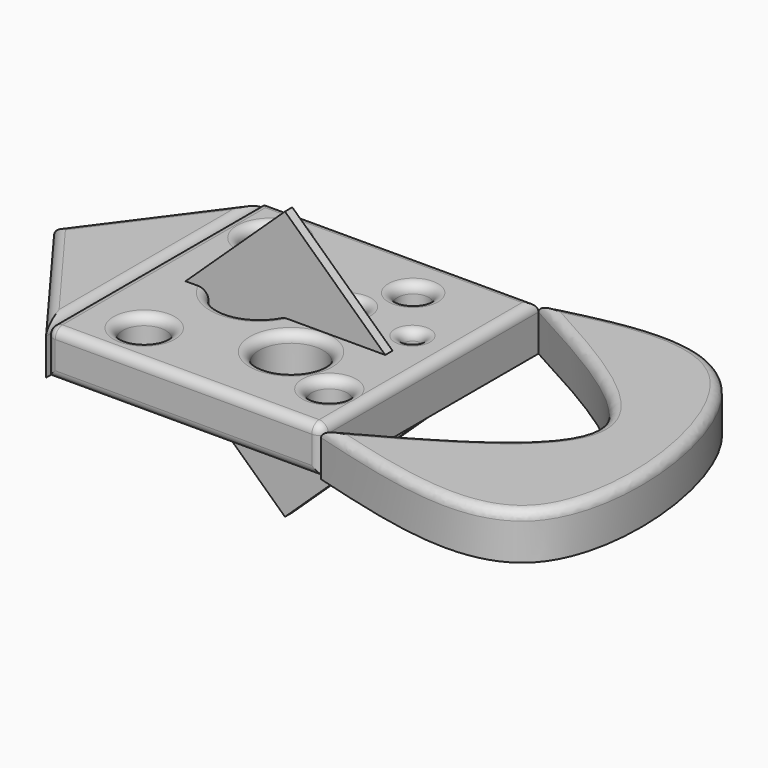
from build123d import *

# Parameters (mm, degrees)
F0_W         = 152.6045948267
F0_H         = 150.9183645248
F0_R         = 11.9309586608
F0_R_2       = 9.9286899081
F0_R_3       = 17.7906163948
F0_R_4       = 22.2629786526
F0_R_5       = 13.4964962962
F0_R_6       = 8.1874520601
F0_R_7       = 4.7131794668
F0_R_8       = 8.6804433709
F1_DEPTH     = 25.4
F3_DEPTH     = 25.4
F5_DEPTH     = 5.08
F6_T1_DEPTH  = 33.02
F6_T3_DEPTH  = 178.0045948267
F6_T5_DEPTH  = 142.4445948267
F6_T7_DEPTH  = 158.5383645248
F6_S11_W     = 5.08
F6_S11_H     = 5.08
F6_T12_DEPTH = 5.08
F6_S17_W     = 5.08
F6_S17_H     = 5.08
F6_T18_DEPTH = 5.08
F7_R         = 5.08
F8_R         = 5.08


# Not quite as in the source:
# - a fillet or chamfer that OpenCascade refuses, or shapes differently, is made with other operations: its cross-section is extruded or revolved along the edge and cut away or added


with BuildPart() as f1:
    # F0 (on Top) → F1 (new body)
    with BuildSketch(Plane.XY):
        Rectangle(F0_W, F0_H)
        with Locations((-41.7344048619, -50.5871586502)):
            Circle(F0_R, mode=Mode.SUBTRACT)
        with Locations((56.7151419818, -45.2293604612)):
            Circle(F0_R_2, mode=Mode.SUBTRACT)
        with Locations((21.9211075455, -28.2444972545)):
            Circle(F0_R_3, mode=Mode.SUBTRACT)
        with Locations((-23.6073378474, 6.744956132)):
            Circle(F0_R_4, mode=Mode.SUBTRACT)
        with Locations((-51.8518351018, 49.7440397739)):
            Circle(F0_R_5, mode=Mode.SUBTRACT)
        with Locations((14.5029760897, 19.8888368905)):
            Circle(F0_R_6, mode=Mode.SUBTRACT)
        with Locations((53.5380840302, 16.4408273995)):
            Circle(F0_R_7, mode=Mode.SUBTRACT)
        with Locations((28.6660604179, 48.0578020215)):
            Circle(F0_R_8, mode=Mode.SUBTRACT)
    extrude(amount=F1_DEPTH)

    # F6: fillet of radius 5.08 on 15 edges, made by hand

    # F6_s2 → F6_t1 (cut)
    with BuildSketch(Plane.XY.offset(-12.7)):
        with BuildLine():
            ThreePointArc((-76.3022974133, -70.3791822624), (-74.8143998618, -73.9712847108), (-71.2222974133, -75.4591822624))
            Line((-71.2222974133, -75.4591822624), (-76.3022974133, -75.4591822624))
            Line((-76.3022974133, -75.4591822624), (-76.3022974133, -70.3791822624))
        make_face()
        with BuildLine():
            ThreePointArc((71.2222974133, -75.4591822624), (74.8143998618, -73.9712847108), (76.3022974133, -70.3791822624))
            Line((76.3022974133, -70.3791822624), (76.3022974133, -75.4591822624))
            Line((76.3022974133, -75.4591822624), (71.2222974133, -75.4591822624))
        make_face()
    extrude(amount=F6_T1_DEPTH, mode=Mode.SUBTRACT)

    # F6_s4 → F6_t3 (cut)
    with BuildSketch(Plane.YZ.offset(-89.0022974133)):
        with BuildLine():
            ThreePointArc((-75.4591822624, 5.08), (-73.9712847108, 1.4878975516), (-70.3791822624, 0))
            Line((-70.3791822624, 0), (-75.4591822624, 0))
            Line((-75.4591822624, 0), (-75.4591822624, 5.08))
        make_face()
        with BuildLine():
            ThreePointArc((75.4591822624, 20.32), (73.9712847108, 23.9121024484), (70.3791822624, 25.4))
            Line((70.3791822624, 25.4), (75.4591822624, 25.4))
            Line((75.4591822624, 25.4), (75.4591822624, 20.32))
        make_face()
    extrude(amount=F6_T3_DEPTH, mode=Mode.SUBTRACT)

    # F6_s6 → F6_t5 (cut)
    with BuildSketch(Plane.YZ.offset(-71.2222974133)):
        with BuildLine():
            ThreePointArc((-75.4591822624, 20.32), (-73.9712847108, 23.9121024484), (-70.3791822624, 25.4))
            Line((-70.3791822624, 25.4), (-75.4591822624, 25.4))
            Line((-75.4591822624, 25.4), (-75.4591822624, 20.32))
        make_face()
    extrude(amount=F6_T5_DEPTH, mode=Mode.SUBTRACT)

    # F6_s8 → F6_t7 (cut)
    with BuildSketch(Plane.XZ.offset(-88.1591822624)):
        with BuildLine():
            ThreePointArc((-76.3022974133, 20.32), (-74.8143998618, 23.9121024484), (-71.2222974133, 25.4))
            Line((-71.2222974133, 25.4), (-76.3022974133, 25.4))
            Line((-76.3022974133, 25.4), (-76.3022974133, 20.32))
        make_face()
        with BuildLine():
            ThreePointArc((76.3022974133, 20.32), (74.8143998618, 23.9121024484), (71.2222974133, 25.4))
            Line((71.2222974133, 25.4), (76.3022974133, 25.4))
            Line((76.3022974133, 25.4), (76.3022974133, 20.32))
        make_face()
    extrude(amount=F6_T7_DEPTH, mode=Mode.SUBTRACT)


with BuildPart() as f3:
    # F2 (on face) → F3 (new body)
    with BuildSketch(Plane.XY.offset(25.4)):
        Polygon((-76.3022974133, -75.4591822624), (-76.3022974133, 75.4591822624), (-132.2656422853, 0), align=None)
    extrude(amount=-F3_DEPTH)

    # F8
    f8_edges = [f3.edges().sort_by_distance(p)[0] for p in [
        (-76.302297, 0, 25.4),
        (-104.28397, 37.729591, 25.4),
        (-104.28397, -37.729591, 25.4),
    ]]
    fillet(f8_edges, radius=F8_R)


with BuildPart() as f3b:
    # F2 (on face) → F3, piece 2 (new body)
    with BuildSketch(Plane.XY.offset(25.4)):
        with BuildLine():
            add(Edge.make_bspline(
                [(76.3022974133, 75.4591822624), (116.4970383218, 85.8497470481), (203.7587624378, 108.4073895966), (233.5011205607, -119.9087985164), (127.2335971306, -89.8605415247), (76.3022974133, -75.4591822624)],
                knots=[0, 0, 0, 0, 0.3078121712, 0.6682521185, 1, 1, 1, 1], degree=3))
            add(Edge.make_bspline(
                [(76.3022974133, 75.4591822624), (122.6474307477, 50.3061215083), (215.3376974165, 0), (122.6474307477, -50.3061215083), (76.3022974133, -75.4591822624)],
                knots=[0, 0, 0, 0, 0.5, 1, 1, 1, 1], degree=3))
        make_face()
    extrude(amount=-F3_DEPTH)

    # F7
    f7_edges = [f3b.edges().sort_by_distance(p)[0] for p in [
        (212.260303, -10.111069, 25.4),
        (168.992564, 0, 25.4),
    ]]
    fillet(f7_edges, radius=F7_R)


with BuildPart() as f5:
    # F4 (on Front) → F5 (new body)
    with BuildSketch(Plane.XZ):
        Polygon((0, 77.4029865861), (-76.8501013517, 4.9759130925), (75.7443532348, 6.6345483065), align=None)
    extrude(amount=F5_DEPTH)


with BuildPart() as f5b:
    # F4 (on Front) → F5, piece 2 (new body)
    with BuildSketch(Plane.XZ):
        Polygon((76.1863735795, 0), (-76.8501013517, 0), (0, -71.8015458847), align=None)
    extrude(amount=F5_DEPTH)


with BuildPart() as f6_tool10:
    # F6_s11 → F6_t12 (new body)
    with BuildSketch(Plane.YZ.offset(-71.2222974133)):
        with Locations((-72.9191822624, 22.86)):
            Rectangle(F6_S11_W, F6_S11_H)
    extrude(amount=-F6_T12_DEPTH)

    # F6_s13 → F6_t14 (revolve, cut)
    with BuildSketch(Plane(origin=(-71.2222974133, -70.3791822624, 20.32), x_dir=(0, 0.7071067812, -0.7071067812), z_dir=(0, 0.7071067812, 0.7071067812))):
        with BuildLine():
            ThreePointArc((0, -5.08), (5.08, 0), (0, 5.08))
            Line((0, 5.08), (0, -5.08))
        make_face()
    revolve(axis=Axis((-71.2222974133, -70.3791822624, 20.32), (-1, 0, 0)), mode=Mode.SUBTRACT)


with BuildPart() as f1_1:
    add(f1.part)

    # F6_t9: cut F6_tool10
    add(f6_tool10.part, mode=Mode.SUBTRACT)


with BuildPart() as f6_tool16:
    # F6_s17 → F6_t18 (new body)
    with BuildSketch(Plane.XZ.offset(70.3791822624)):
        with Locations((73.7622974133, 22.86)):
            Rectangle(F6_S17_W, F6_S17_H)
    extrude(amount=F6_T18_DEPTH)

    # F6_s19 → F6_t20 (revolve, cut)
    with BuildSketch(Plane(origin=(71.2222974133, -70.3791822624, 20.32), x_dir=(-0.7071067812, 0, -0.7071067812), z_dir=(-0.7071067812, 0, 0.7071067812))):
        with BuildLine():
            ThreePointArc((0, -5.08), (5.08, 0), (0, 5.08))
            Line((0, 5.08), (0, -5.08))
        make_face()
    revolve(axis=Axis((71.2222974133, -70.3791822624, 20.32), (0, -1, 0)), mode=Mode.SUBTRACT)


with BuildPart() as f1_2:
    add(f1_1.part)

    # F6_t15: cut F6_tool16
    add(f6_tool16.part, mode=Mode.SUBTRACT)

    # F6_s21 → F6_t22 (revolve, cut)
    with BuildSketch(Plane.XZ.offset(50.5871586502)):
        with BuildLine():
            ThreePointArc((-29.8034462012, 20.32), (-28.3155486496, 23.9121024484), (-24.7234462012, 25.4))
            Line((-24.7234462012, 25.4), (-29.8034462012, 25.4))
            Line((-29.8034462012, 25.4), (-29.8034462012, 20.32))
        make_face()
    revolve(axis=Axis((-41.7344048619, -50.5871586502, 25.4), (0, 0, 1)), mode=Mode.SUBTRACT)

    # F6_s23 → F6_t24 (revolve, cut)
    with BuildSketch(Plane.XZ.offset(45.2293604612)):
        with BuildLine():
            ThreePointArc((66.6438318899, 20.32), (68.1317294415, 23.9121024484), (71.7238318899, 25.4))
            Line((71.7238318899, 25.4), (66.6438318899, 25.4))
            Line((66.6438318899, 25.4), (66.6438318899, 20.32))
        make_face()
    revolve(axis=Axis((56.7151419818, -45.2293604612, 25.4), (0, 0, 1)), mode=Mode.SUBTRACT)

    # F6_s25 → F6_t26 (revolve, cut)
    with BuildSketch(Plane.XZ.offset(28.2444972545)):
        with BuildLine():
            ThreePointArc((39.7117239403, 20.32), (41.1996214919, 23.9121024484), (44.7917239403, 25.4))
            Line((44.7917239403, 25.4), (39.7117239403, 25.4))
            Line((39.7117239403, 25.4), (39.7117239403, 20.32))
        make_face()
    revolve(axis=Axis((21.9211075455, -28.2444972545, 25.4), (0, 0, 1)), mode=Mode.SUBTRACT)

    # F6_s27 → F6_t28 (revolve, cut)
    with BuildSketch(Plane.XZ.offset(-6.744956132)):
        with BuildLine():
            ThreePointArc((-1.3443591948, 20.32), (0.1435383568, 23.9121024484), (3.7356408052, 25.4))
            Line((3.7356408052, 25.4), (-1.3443591948, 25.4))
            Line((-1.3443591948, 25.4), (-1.3443591948, 20.32))
        make_face()
    revolve(axis=Axis((-23.6073378474, 6.744956132, 25.4), (0, 0, 1)), mode=Mode.SUBTRACT)

    # F6_s29 → F6_t30 (revolve, cut)
    with BuildSketch(Plane.XZ.offset(-49.7440397739)):
        with BuildLine():
            ThreePointArc((-38.3553388057, 20.32), (-36.8674412541, 23.9121024484), (-33.2753388057, 25.4))
            Line((-33.2753388057, 25.4), (-38.3553388057, 25.4))
            Line((-38.3553388057, 25.4), (-38.3553388057, 20.32))
        make_face()
    revolve(axis=Axis((-51.8518351018, 49.7440397739, 25.4), (0, 0, 1)), mode=Mode.SUBTRACT)

    # F6_s31 → F6_t32 (revolve, cut)
    with BuildSketch(Plane.XZ.offset(-19.8888368905)):
        with BuildLine():
            ThreePointArc((22.6904281498, 20.32), (24.1783257014, 23.9121024484), (27.7704281498, 25.4))
            Line((27.7704281498, 25.4), (22.6904281498, 25.4))
            Line((22.6904281498, 25.4), (22.6904281498, 20.32))
        make_face()
    revolve(axis=Axis((14.5029760897, 19.8888368905, 25.4), (0, 0, 1)), mode=Mode.SUBTRACT)

    # F6_s33 → F6_t34 (revolve, cut)
    with BuildSketch(Plane.XZ.offset(-16.4408273995)):
        with BuildLine():
            ThreePointArc((58.251263497, 20.32), (59.7391610486, 23.9121024484), (63.331263497, 25.4))
            Line((63.331263497, 25.4), (58.251263497, 25.4))
            Line((58.251263497, 25.4), (58.251263497, 20.32))
        make_face()
    revolve(axis=Axis((53.5380840302, 16.4408273995, 25.4), (0, 0, 1)), mode=Mode.SUBTRACT)

    # F6_s35 → F6_t36 (revolve, cut)
    with BuildSketch(Plane.XZ.offset(-48.0578020215)):
        with BuildLine():
            ThreePointArc((37.3465037888, 20.32), (38.8344013404, 23.9121024484), (42.4265037888, 25.4))
            Line((42.4265037888, 25.4), (37.3465037888, 25.4))
            Line((37.3465037888, 25.4), (37.3465037888, 20.32))
        make_face()
    revolve(axis=Axis((28.6660604179, 48.0578020215, 25.4), (0, 0, 1)), mode=Mode.SUBTRACT)


solid = Compound([f3.part, f3b.part, f5.part, f5b.part, f1_2.part])
